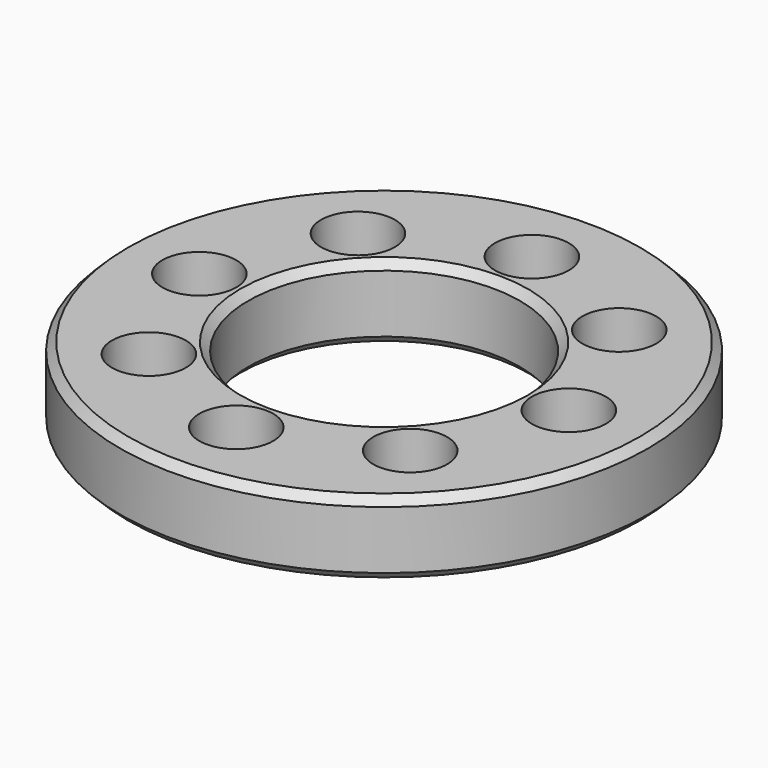
from build123d import *

# Parameters (mm, degrees)
F0_R            = 10
F0_R_2          = 5.15
F1_DEPTH        = 2.8
F3_D            = 2.8
F3_COPIES_COUNT = 8
F4_SIZE         = 0.3


# Not quite as in the source:
# - a pattern or mirror of a feature is missing from the dataset's text; its kind, count and spacing are read off the source's solid


with BuildPart() as f1:
    # F0 (on Top) → F1 (new body)
    with BuildSketch(Plane.XY):
        Circle(F0_R)
        Circle(F0_R_2, mode=Mode.SUBTRACT)
    extrude(amount=F1_DEPTH)

    # F3 (through all)
    with Locations(Plane.XY.offset(2.8)):
        with Locations((0, 7)):
            f3 = Hole(F3_D / 2)

    # F3_copies: F3 ×8 about axis
    f3_copies_axis = Axis((0, 0, 0), (0, 0, 1))
    for i in range(1, F3_COPIES_COUNT):
        add(f3.rotate(f3_copies_axis, i * 360 / F3_COPIES_COUNT), mode=Mode.SUBTRACT)

    # F4
    f4_edges = [f1.edges().sort_by_distance(p)[0] for p in [
        (-5.15, 0, 0),
        (-10, 0, 0),
        (-5.15, 0, 2.8),
        (-10, 0, 2.8),
    ]]
    chamfer(f4_edges, length=F4_SIZE)


solid = f1.part
